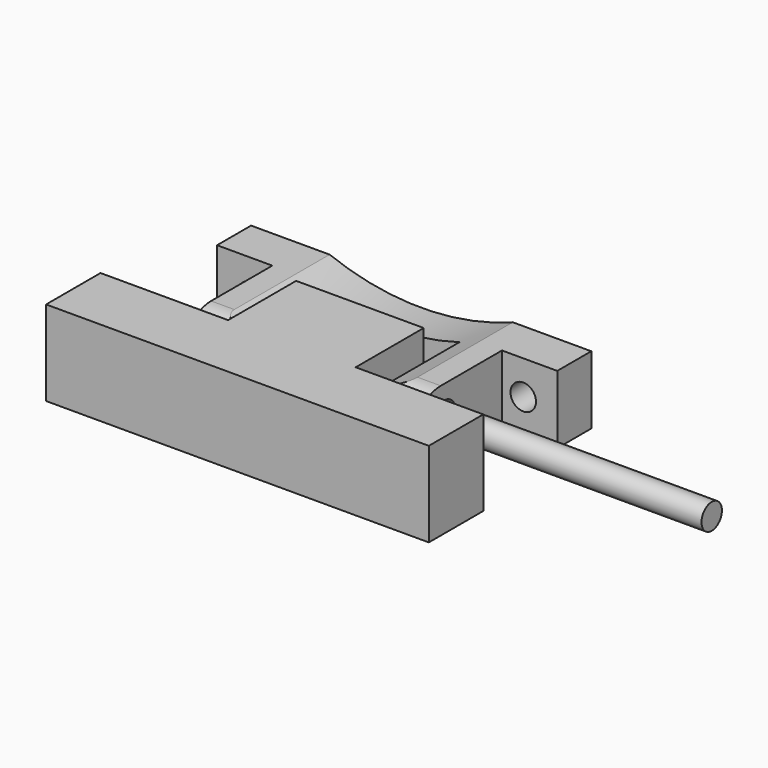
from build123d import *

# Parameters (mm, degrees)
F1_DEPTH  = 10
F2_DEPTH  = 8
F3_R      = 1.75
F4_DEPTH  = 50
F5_R      = 1.5
F6_DEPTH  = 25
F7_DEPTH  = 1
F8_R      = 4
F9_R      = 1.5
F10_DEPTH = 16.3613527737


with BuildPart() as f1:
    # F0 (on Top) → F1 (new body)
    with BuildSketch(Plane.XY):
        Polygon((15, 0), (0, 0), (0, -10), (-15, -10), (-15, -18), (30, -18), (30, -10), (15, -10), align=None)
    extrude(amount=F1_DEPTH)


with BuildPart() as f2:
    # F0 (on Top) → F2 (new body)
    with BuildSketch(Plane.XY):
        Polygon((-6, 4), (-6, -9), (-1, -9), (-1, 4), (16, 4), (16, -9), (21, -9), (21, 4), (23.5, 4), (27.5, 4), (27.5, 9), (-12.5, 9), (-12.5, 4), (-8.5, 4), align=None)
        with BuildLine():
            ThreePointArc((-7, 5.5), (-7.4393398282, 4.4393398282), (-8.5, 4))
            ThreePointArc((-8.5, 4), (-9.5606601718, 6.5606601718), (-7, 5.5))
        make_face(mode=Mode.SUBTRACT)
        with BuildLine():
            ThreePointArc((25, 5.5), (24.5606601718, 4.4393398282), (23.5, 4))
            ThreePointArc((23.5, 4), (22.4393398282, 6.5606601718), (25, 5.5))
        make_face(mode=Mode.SUBTRACT)
        with BuildLine():
            ThreePointArc((-7, 5.5), (-9.5606601718, 6.5606601718), (-8.5, 4))
            ThreePointArc((-8.5, 4), (-7.4393398282, 4.4393398282), (-7, 5.5))
        make_face()
        with BuildLine():
            ThreePointArc((25, 5.5), (22.4393398282, 6.5606601718), (23.5, 4))
            ThreePointArc((23.5, 4), (24.5606601718, 4.4393398282), (25, 5.5))
        make_face()
    extrude(amount=F2_DEPTH)


with BuildPart() as f4_tool:
    # F3 (on face) → F4 (new body, symmetric)
    with BuildSketch(Plane(origin=(0, 0, 0), x_dir=(0, -1, 0), z_dir=(-1, 0, 0))):
        with Locations((4.55, 4.55)):
            Circle(F3_R)
    extrude(amount=F4_DEPTH, both=True)


with BuildPart() as f1_1:
    add(f1.part)

    # F4: cut by f4_tool
    add(f4_tool.part, mode=Mode.SUBTRACT)

    # F0 (on Top) → F7 (cut)
    with BuildSketch(Plane.XY):
        Polygon((-12.5, 4), (-12.5, -9), (-6, -9), (-6, 4), (-8.5, 4), align=None)
    extrude(amount=F7_DEPTH, mode=Mode.SUBTRACT)


with BuildPart() as f2_1:
    add(f2.part)

    # F4: cut by f4_tool
    add(f4_tool.part, mode=Mode.SUBTRACT)

    # F8
    f8_edges = [f2_1.edges().sort_by_distance(p)[0] for p in [
        (18.5, -9, 8),
        (-3.5, -9, 8),
    ]]
    fillet(f8_edges, radius=F8_R)

    # F9 (on face) → F10 (cut, through all)
    with BuildSketch(Plane(origin=(0, 9, 0), x_dir=(-1, 0, 0), z_dir=(0, 1, 0))):
        with Locations((8.5, 4)):
            Circle(F9_R)
        with Locations((-23.5, 4)):
            Circle(F9_R)
        with BuildLine():
            Line((3.2703296143, 8), (-18.2703296143, 8))
            ThreePointArc((-18.2703296143, 8), (-7.5, 6), (3.2703296143, 8))
        make_face()
    extrude(amount=-F10_DEPTH, mode=Mode.SUBTRACT)


with BuildPart() as f6:
    # F5 (on face) → F6 (new body, symmetric)
    with BuildSketch(Plane.YZ.offset(27.5)):
        with Locations((-4.55, 4.55)):
            Circle(F5_R)
    extrude(amount=F6_DEPTH, both=True)


solid = Compound([f1_1.part, f2_1.part, f6.part])
